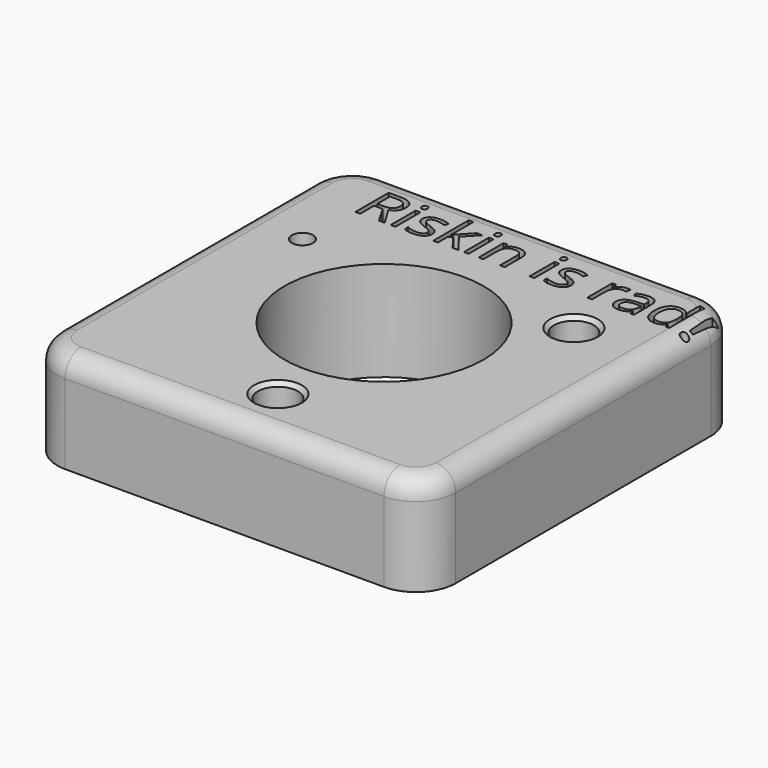
from build123d import *

# Parameters (mm, degrees)
F0_R         = 5
F0_R_2       = 25
F0_R_3       = 2.6684569823
F1_DEPTH     = 12.5
F2_TEXT_SIZE = 14.6345278142
F3_DEPTH     = 5
F4_T1_DEPTH  = 80
F4_T3_DEPTH  = 80
F4_T6_ANGLE  = 90
F4_T8_ANGLE  = 90
F4_T10_ANGLE = 90
F4_T12_ANGLE = 90
F5_SIZE      = 1


# Not quite as in the source:
# - a fillet or chamfer that OpenCascade refuses, or shapes differently, is made with other operations: its cross-section is extruded or revolved along the edge and cut away or added
# - Text() gives the source's letters only with a copy of the font that has no kerning and outlines rounded to 1/6400 em; it was checked with that copy


with BuildPart() as f1:
    # F0 (on Top) → F1 (new body, symmetric)
    with BuildSketch(Plane.XY):
        with BuildLine():
            Line((40, 50), (-40, 50))
            ThreePointArc((-40, 50), (-47.0710678119, 47.0710678119), (-50, 40))
            Line((-50, 40), (-50, -40))
            ThreePointArc((-50, -40), (-47.0710678119, -47.0710678119), (-40, -50))
            Line((-40, -50), (40, -50))
            ThreePointArc((40, -50), (47.0710678119, -47.0710678119), (50, -40))
            Line((50, -40), (50, 40))
            ThreePointArc((50, 40), (47.0710678119, 47.0710678119), (40, 50))
        make_face()
        with Locations((2.6294370182, -36.5616902709)):
            Circle(F0_R, mode=Mode.SUBTRACT)
        with Locations((-34.683521837, 17.7800003439)):
            Circle(F0_R, mode=Mode.SUBTRACT)
        Circle(F0_R_2, mode=Mode.SUBTRACT)
        with Locations((30.4263364524, 21.5363390744)):
            Circle(F0_R, mode=Mode.SUBTRACT)
        with Locations((-34.683521837, 17.7800003439)):
            Circle(F0_R)
        with Locations((-34.683521837, 17.7800003439)):
            Circle(F0_R_3, mode=Mode.SUBTRACT)
    extrude(amount=F1_DEPTH, both=True)

    # F2 (on face) → F3 (cut)
    with BuildSketch(Plane.XY.offset(12.5)):
        with Locations((-35.2209714229, 33.2470825564)):
            Text('Riskin is rad!', F2_TEXT_SIZE, font='Open Sans', text_align=(TextAlign.LEFT, TextAlign.BOTTOM))
    extrude(amount=-F3_DEPTH, mode=Mode.SUBTRACT)

    # F4: fillet of radius 5 on 8 edges, made by hand

    # F4_s2 → F4_t1 (cut)
    with BuildSketch(Plane.XZ.offset(-40)):
        with BuildLine():
            ThreePointArc((-45, 12.5), (-48.5355339059, 11.0355339059), (-50, 7.5))
            Line((-50, 7.5), (-50, 12.5))
            Line((-50, 12.5), (-45, 12.5))
        make_face()
        with BuildLine():
            ThreePointArc((45, 12.5), (48.5355339059, 11.0355339059), (50, 7.5))
            Line((50, 7.5), (50, 12.5))
            Line((50, 12.5), (45, 12.5))
        make_face()
    extrude(amount=F4_T1_DEPTH, mode=Mode.SUBTRACT)

    # F4_s4 → F4_t3 (cut)
    with BuildSketch(Plane.YZ.offset(-40)):
        with BuildLine():
            ThreePointArc((50, 7.5), (48.5355339059, 11.0355339059), (45, 12.5))
            Line((45, 12.5), (50, 12.5))
            Line((50, 12.5), (50, 7.5))
        make_face()
        with BuildLine():
            ThreePointArc((-45, 12.5), (-48.5355339059, 11.0355339059), (-50, 7.5))
            Line((-50, 7.5), (-50, 12.5))
            Line((-50, 12.5), (-45, 12.5))
        make_face()
    extrude(amount=F4_T3_DEPTH, mode=Mode.SUBTRACT)

    # F4_s5 → F4_t6 (revolve, cut)
    with BuildSketch(Plane.YZ.offset(-40)):
        with BuildLine():
            ThreePointArc((50, 7.5), (48.5355339059, 11.0355339059), (45, 12.5))
            Line((45, 12.5), (50, 12.5))
            Line((50, 12.5), (50, 7.5))
        make_face()
    revolve(axis=Axis((-40, 40, 12.5), (0, 0, 1)), revolution_arc=F4_T6_ANGLE, mode=Mode.SUBTRACT)

    # F4_s7 → F4_t8 (revolve, cut)
    with BuildSketch(Plane.XZ.offset(-40)):
        with BuildLine():
            ThreePointArc((45, 12.5), (48.5355339059, 11.0355339059), (50, 7.5))
            Line((50, 7.5), (50, 12.5))
            Line((50, 12.5), (45, 12.5))
        make_face()
    revolve(axis=Axis((40, 40, 12.5), (0, 0, 1)), revolution_arc=F4_T8_ANGLE, mode=Mode.SUBTRACT)

    # F4_s9 → F4_t10 (revolve, cut)
    with BuildSketch(Plane.YZ.offset(40)):
        with BuildLine():
            ThreePointArc((-45, 12.5), (-48.5355339059, 11.0355339059), (-50, 7.5))
            Line((-50, 7.5), (-50, 12.5))
            Line((-50, 12.5), (-45, 12.5))
        make_face()
    revolve(axis=Axis((40, -40, 12.5), (0, 0, 1)), revolution_arc=F4_T10_ANGLE, mode=Mode.SUBTRACT)

    # F4_s11 → F4_t12 (revolve, cut)
    with BuildSketch(Plane.XZ.offset(40)):
        with BuildLine():
            ThreePointArc((-45, 12.5), (-48.5355339059, 11.0355339059), (-50, 7.5))
            Line((-50, 7.5), (-50, 12.5))
            Line((-50, 12.5), (-45, 12.5))
        make_face()
    revolve(axis=Axis((-40, -40, 12.5), (0, 0, 1)), revolution_arc=F4_T12_ANGLE, mode=Mode.SUBTRACT)

    # F5
    f5_edges = [f1.edges().sort_by_distance(p)[0] for p in [
        (25.426336, 21.536339, 12.5),
        (-2.370563, -36.56169, 12.5),
    ]]
    chamfer(f5_edges, length=F5_SIZE)


solid = f1.part
